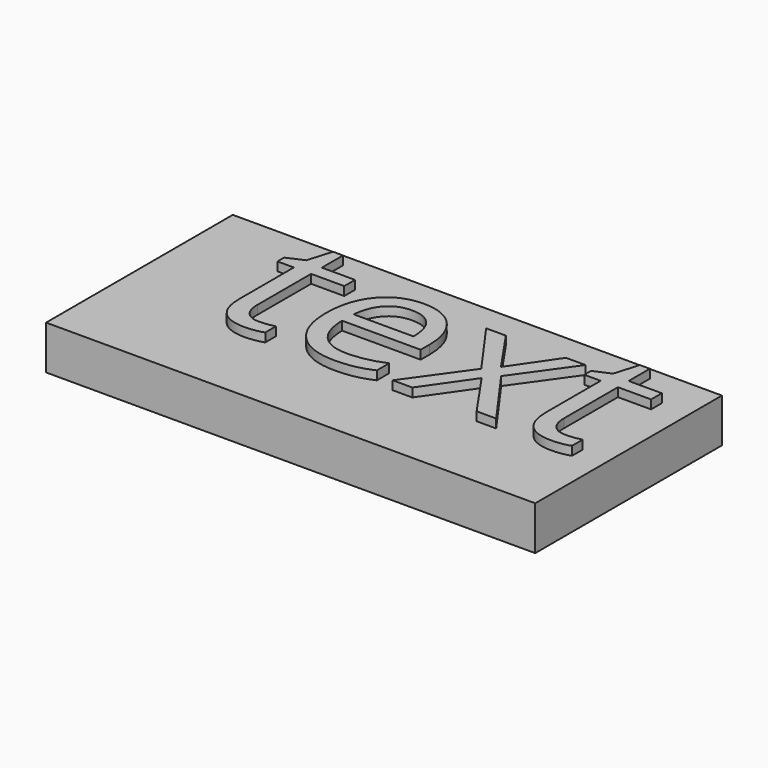
from build123d import *

# Parameters (mm, degrees)
F0_W         = 111.3926805556
F0_H         = 53.1410835683
F1_DEPTH     = 10
F2_TEXT_SIZE = 48.5871297618
F3_DEPTH     = 2


# Not quite as in the source:
# - Text() gives the source's letters only with a copy of the font that has no kerning and outlines rounded to 1/6400 em; it was checked with that copy


with BuildPart() as f1:
    # F0 (on Top) → F1 (new body)
    with BuildSketch(Plane.XY):
        with Locations((-0.3450382501, 8.4121916443)):
            Rectangle(F0_W, F0_H)
    extrude(amount=F1_DEPTH)

    # F2 (on face) → F3 (join)
    with BuildSketch(Plane.XY.offset(10)):
        with Locations((-36.9639508426, 0)):
            Text('text', F2_TEXT_SIZE, font='Open Sans', text_align=(TextAlign.LEFT, TextAlign.BOTTOM))
    extrude(amount=F3_DEPTH)


solid = f1.part
